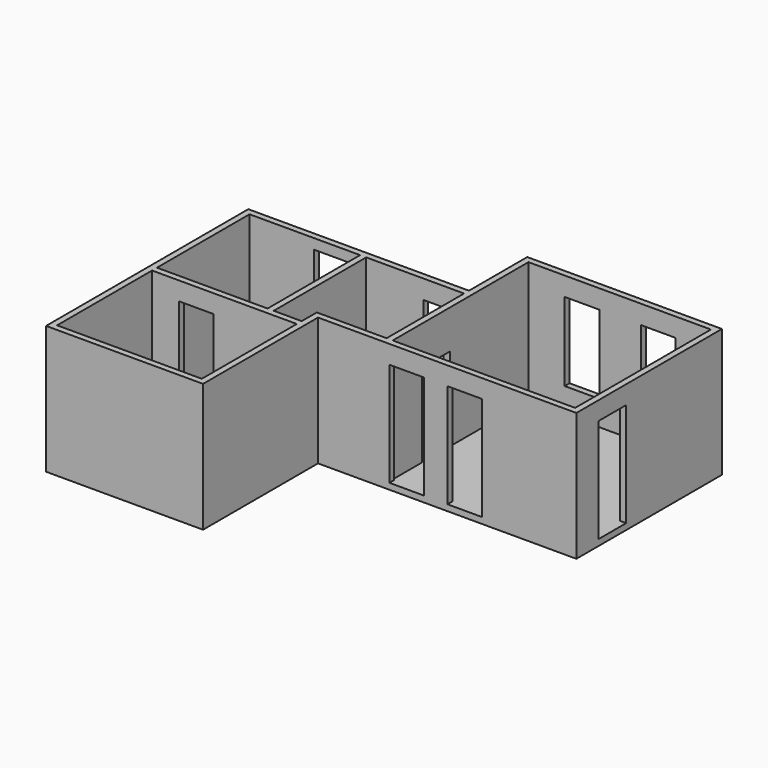
from build123d import *

# Parameters (mm, degrees)
F1_DEPTH  = 3048
F3_DEPTH  = 152.4
F4_W      = 863.6
F4_H      = 2590.8
F5_DEPTH  = 3733.801
F6_W      = 863.6
F6_H      = 1955.8
F7_DEPTH  = 152.401
F8_W      = 863.6
F8_H      = 2590.8
F9_DEPTH  = 152.401
F10_W     = 152.4
F10_H     = 2413
F10_W_2   = 3606.8
F10_H_2   = 152.4
F11_DEPTH = 3048
F12_W     = 609.6
F12_H     = 1955.8
F12_W_2   = 863.6
F12_H_2   = 1473.2
F13_DEPTH = 1968.501
F14_W     = 152.4
F14_H     = 2882.9
F15_DEPTH = 3048
F16_W     = 863.6
F16_H     = 2082.8
F17_DEPTH = 152.4
F18_W     = 863.6
F18_H     = 2590.8
F19_DEPTH = 152.4
F20_W     = 863.6
F20_H     = 2082.8
F21_DEPTH = 152.4
F23_DEPTH = 609.6


with BuildPart() as f1:
    # F0 (on Top) → F1 (new body)
    with BuildSketch(Plane.XY):
        Polygon((152.4, 152.4), (-4699, 152.4), (-4699, -1663.7), (-10198.1, -1663.7), (-10198.1, -7962.9), (-6286.5, -7962.9), (-6286.5, -4381.5), (152.4, -4381.5), align=None)
        Polygon((-4546.6, 0), (0, 0), (0, -4229.1), (-6438.9, -4229.1), (-6438.9, -7810.5), (-10045.7, -7810.5), (-10045.7, -1816.1), (-4546.6, -1816.1), align=None, mode=Mode.SUBTRACT)
    extrude(amount=F1_DEPTH)

    # F2 (on face) → F3 (join)
    with BuildSketch(Plane(origin=(0, 0, 0), x_dir=(1, 0, 0), z_dir=(0, 0, -1))):
        Polygon((-6286.5, 7962.9), (-10198.1, 7962.9), (-10198.1, 1663.7), (-4699, 1663.7), (-4699, -152.4), (152.4, -152.4), (152.4, 4381.5), (-6286.5, 4381.5), align=None)
    extrude(amount=F3_DEPTH)

    # F4 (on face) → F5 (cut, through all)
    with BuildSketch(Plane(origin=(0, -4229.1, 0), x_dir=(-1, 0, 0), z_dir=(0, 1, 0))):
        with Locations((2628.9, 1295.4)):
            Rectangle(F4_W, F4_H)
        with Locations((4076.7, 1295.4)):
            Rectangle(F4_W, F4_H)
    extrude(amount=-F5_DEPTH, mode=Mode.SUBTRACT)

    # F6 (on face) → F7 (cut, through all)
    with BuildSketch(Plane.XZ):
        with Locations((-3213.1, 1600.2)):
            Rectangle(F6_W, F6_H)
        with Locations((-1308.1, 1600.2)):
            Rectangle(F6_W, F6_H)
    extrude(amount=-F7_DEPTH, mode=Mode.SUBTRACT)

    # F8 (on face) → F9 (cut, through all)
    with BuildSketch(Plane(origin=(0, 0, 0), x_dir=(0, -1, 0), z_dir=(-1, 0, 0))):
        with Locations((3263.9, 1295.4)):
            Rectangle(F8_W, F8_H)
    extrude(amount=-F9_DEPTH, mode=Mode.SUBTRACT)

    # F10 (on face) → F11 (join, through all)
    with BuildSketch(Plane.XY):
        with Locations((-4622.8, -3022.6)):
            Rectangle(F10_W, F10_H)
        with Locations((-8242.3, -4775.2)):
            Rectangle(F10_W_2, F10_H_2)
    extrude(amount=F11_DEPTH)

    # F12 (on face) → F13 (cut, through all)
    with BuildSketch(Plane.XZ.offset(1816.1)):
        with Locations((-5410.2, 1600.2)):
            Rectangle(F12_W, F12_H)
        with Locations((-8001, 2057.4)):
            Rectangle(F12_W_2, F12_H_2)
    extrude(amount=-F13_DEPTH, mode=Mode.SUBTRACT)

    # F14 (on face) → F15 (join, through all)
    with BuildSketch(Plane.XY):
        with Locations((-7213.6, -3257.55)):
            Rectangle(F14_W, F14_H)
    extrude(amount=F15_DEPTH)

    # F16 (on face) → F17 (cut, through all)
    with BuildSketch(Plane.YZ.offset(-4546.6)):
        with Locations((-2882.9, 1041.4)):
            Rectangle(F16_W, F16_H)
    extrude(amount=-F17_DEPTH, mode=Mode.SUBTRACT)

    # F18 (on face) → F19 (cut, through all)
    with BuildSketch(Plane(origin=(0, -4699, 0), x_dir=(-1, 0, 0), z_dir=(0, 1, 0))):
        with Locations((8940.8, 1295.4)):
            Rectangle(F18_W, F18_H)
    extrude(amount=-F19_DEPTH, mode=Mode.SUBTRACT)

    # F20 (on face) → F21 (cut, through all)
    with BuildSketch(Plane(origin=(-7289.8, 0, 0), x_dir=(0, -1, 0), z_dir=(-1, 0, 0))):
        with Locations((3257.55, 1041.4)):
            Rectangle(F20_W, F20_H)
    extrude(amount=-F21_DEPTH, mode=Mode.SUBTRACT)

    # F22 (on face) → F23 (join)
    with BuildSketch(Plane.XY):
        with BuildLine():
            ThreePointArc((-6299.2, -3898.9), (-6224.8051224214, -4078.5051224214), (-6045.2, -4152.9))
            Line((-6045.2, -4152.9), (-5029.2, -4152.9))
            ThreePointArc((-5029.2, -4152.9), (-4849.5948775786, -4078.5051224214), (-4775.2, -3898.9))
            Line((-4775.2, -3898.9), (-4775.2, -3644.9))
            ThreePointArc((-4775.2, -3644.9), (-4849.5948775786, -3465.2948775786), (-5029.2, -3390.9))
            Line((-5029.2, -3390.9), (-6045.2, -3390.9))
            ThreePointArc((-6045.2, -3390.9), (-6224.8051224214, -3465.2948775786), (-6299.2, -3644.9))
            Line((-6299.2, -3644.9), (-6299.2, -3898.9))
        make_face()
    extrude(amount=F23_DEPTH)


solid = f1.part
